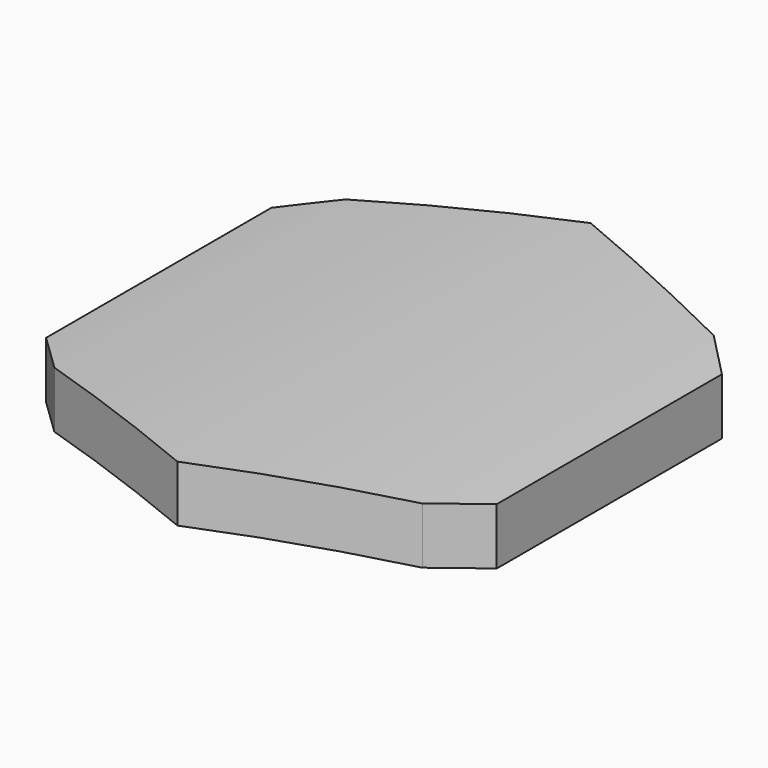
from build123d import *

# Parameters (mm, degrees)
F1_DEPTH    = 10
F2_SIZE     = 2.5
F3_T1_DEPTH = 13.9641748973


# Not quite as in the source:
# - a fillet or chamfer that OpenCascade refuses, or shapes differently, is made with other operations: its cross-section is extruded or revolved along the edge and cut away or added


with BuildPart() as f1:
    # F0 (on Front) → F1 (new body)
    with BuildSketch(Plane.XZ):
        with BuildLine():
            Line((4, 36.2801598673), (4, 37.286056375))
            ThreePointArc((4, 37.286056375), (0, 37.5), (-4, 37.286056375))
            Line((-4, 37.286056375), (-4, 36.2801598673))
            ThreePointArc((-4, 36.2801598673), (0, 36.5), (4, 36.2801598673))
        make_face()
    extrude(amount=F1_DEPTH)

    # F2
    f2_edges = [f1.edges().sort_by_distance(p)[0] for p in [
        (-4, -10, 36.783108),
        (-4, 0, 36.783108),
        (4, 0, 36.783108),
        (4, -10, 36.783108),
    ]]
    chamfer(f2_edges, length=F2_SIZE)

    # F3: chamfer of 2.5 on 4 edges, made by hand

    # F3_s2 → F3_t1 (cut)
    with BuildSketch(Plane.XY.offset(29.9874890754)):
        Polygon((-3.267766953, -8.232233047), (1, -10), (-1.5, -10), align=None)
        Polygon((-1, -10), (3.267766953, -8.232233047), (1.5, -10), align=None)
        Polygon((-3.267766953, -1.767766953), (1, 0), (-1.5, 0), align=None)
        Polygon((-1, 0), (3.267766953, -1.767766953), (1.5, 0), align=None)
    extrude(amount=F3_T1_DEPTH, mode=Mode.SUBTRACT)


solid = f1.part
